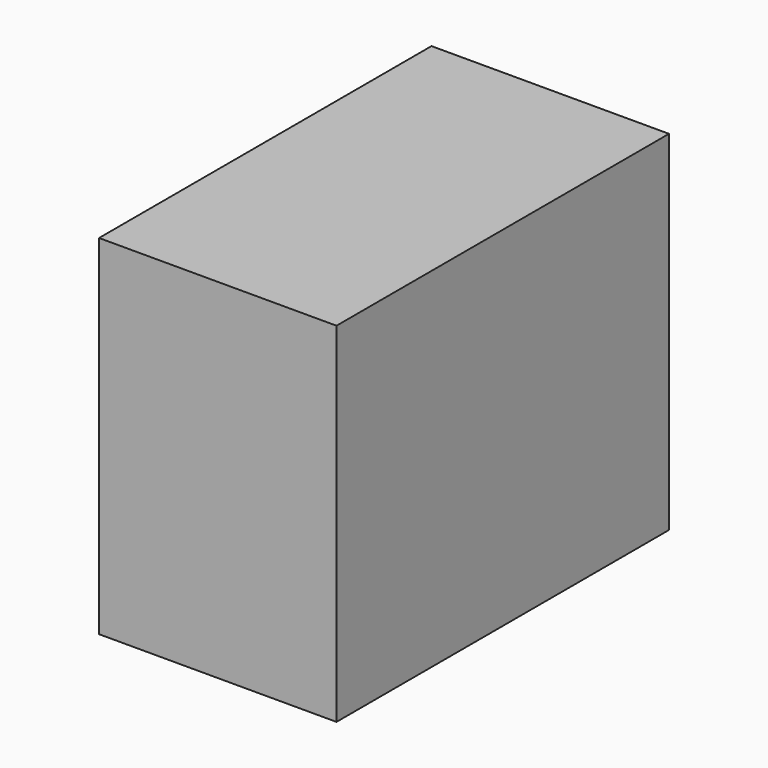
from build123d import *

# Parameters (mm, degrees)
F1_W     = 101.6
F1_H     = 177.8
F1_W_2   = 38.1
F1_H_2   = 48.6833333333
F1_H_3   = 158.75
F2_DEPTH = 139.7
F3_W     = 101.6
F3_H     = 177.8
F4_DEPTH = 9.525


# Not quite as in the source:
# - a variable given as a bare number and used for a length is read in inches; the dataset says mm whatever the document's units were


with BuildPart() as f2:
    # F1 (on Top) → F2 (new body)
    with BuildSketch(Plane.XY):
        with Locations((50.8, 88.9)):
            Rectangle(F1_W, F1_H)
        with Locations((28.575, 33.8666666667)):
            Rectangle(F1_W_2, F1_H_2, mode=Mode.SUBTRACT)
        with Locations((28.575, 88.9)):
            Rectangle(F1_W_2, F1_H_2, mode=Mode.SUBTRACT)
        with Locations((28.575, 143.9333333333)):
            Rectangle(F1_W_2, F1_H_2, mode=Mode.SUBTRACT)
        with Locations((73.025, 88.9)):
            Rectangle(F1_W_2, F1_H_3, mode=Mode.SUBTRACT)
    extrude(amount=F2_DEPTH)

    # F3 (on face) → F4 (join)
    with BuildSketch(Plane.XY.offset(139.7)):
        with Locations((50.8, 88.9)):
            Rectangle(F3_W, F3_H)
    extrude(amount=F4_DEPTH)


solid = f2.part
